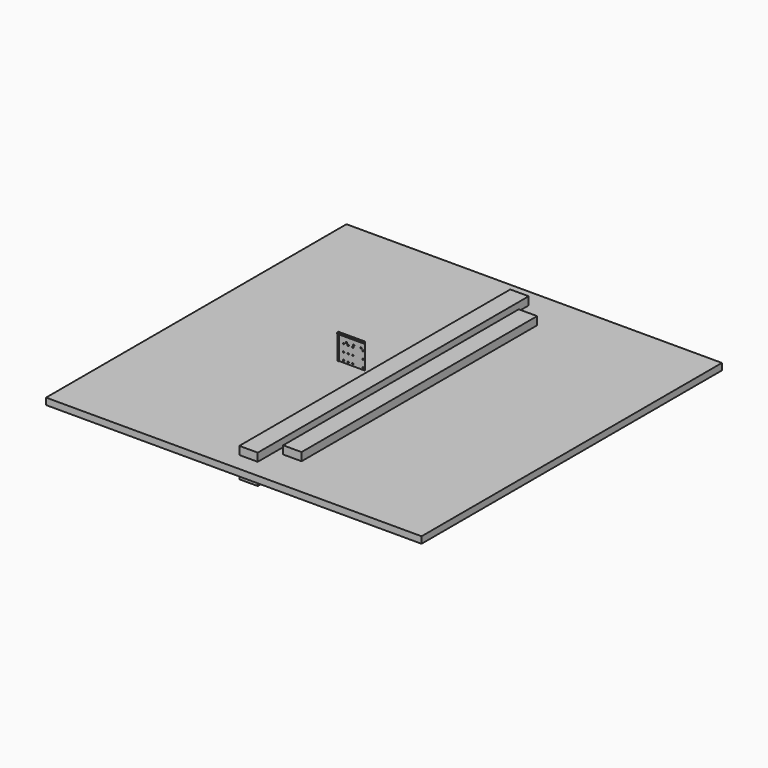
from build123d import *

# Parameters (mm, degrees)
F0_W     = 50
F0_H     = 80
F1_DEPTH = 460
F2_DEPTH = 400
F3_R     = 1.85
F3_W     = 2.75
F3_H     = 65.8975437433
F3_W_2   = 20.0489750504
F3_H_2   = 2.75
F4_DEPTH = 1.5
F5_DEPTH = 5
F6_DEPTH = 3.5
F7_W     = 1020
F7_H     = 1020
F8_DEPTH = 18


with BuildPart() as f1:
    # F0 (on Front) → F1 (new body, symmetric)
    with BuildSketch(Plane.XZ):
        Rectangle(F0_W, F0_H)
    extrude(amount=F1_DEPTH, both=True)


with BuildPart() as f2:
    # F0 (on Front) → F2 (new body, symmetric)
    with BuildSketch(Plane.XZ):
        with Locations((71.0044652224, 0)):
            Rectangle(F0_W, F0_H)
    extrude(amount=F2_DEPTH, both=True)


with BuildPart() as f4:
    # F3 (on Front) → F4 (new body)
    with BuildSketch(Plane.XZ):
        Polygon((-121.2795429826, 25.1443590969), (-71.0295429826, 25.1443590969), (-71.0295429826, 90.7919028401), (-71.0295429826, 91.0419028401), (-121.2795429826, 91.0419028401), align=None)
        with Locations((-108.5295429826, 30.7919028401)):
            Circle(F3_R, mode=Mode.SUBTRACT)
        with Locations((-96.0295429826, 30.7919028401)):
            Circle(F3_R, mode=Mode.SUBTRACT)
        with Locations((-108.5295429826, 50.7919028401)):
            Circle(F3_R, mode=Mode.SUBTRACT)
        with Locations((-96.0295429826, 50.7919028401)):
            Circle(F3_R, mode=Mode.SUBTRACT)
        with Locations((-83.5295429826, 30.7919028401)):
            Circle(F3_R, mode=Mode.SUBTRACT)
        with Locations((-83.5295429826, 50.7919028401)):
            Circle(F3_R, mode=Mode.SUBTRACT)
        with Locations((-108.5295429826, 70.7919028401)):
            Circle(F3_R, mode=Mode.SUBTRACT)
        with Locations((-101.0295429826, 75.7919028401)):
            Circle(F3_R, mode=Mode.SUBTRACT)
        with Locations((-96.0295429826, 70.7919028401)):
            Circle(F3_R, mode=Mode.SUBTRACT)
        with Locations((-83.5295429826, 70.7919028401)):
            Circle(F3_R, mode=Mode.SUBTRACT)
        with Locations((-81.0295429826, 75.7919028401)):
            Circle(F3_R, mode=Mode.SUBTRACT)
        Polygon((-71.0295429826, 90.7919028401), (-71.0295429826, 25.1443590969), (-50.9805679321, 25.1443590969), (-50.9805679321, 91.0419028401), (-71.0295429826, 91.0419028401), align=None)
        with Locations((-56.0295429826, 30.3744599223)):
            Circle(F3_R, mode=Mode.SUBTRACT)
        with Locations((-56.0295429826, 50.7919028401)):
            Circle(F3_R, mode=Mode.SUBTRACT)
        with Locations((-61.0295429826, 75.7919028401)):
            Circle(F3_R, mode=Mode.SUBTRACT)
        with Locations((-56.0295429826, 70.7919028401)):
            Circle(F3_R, mode=Mode.SUBTRACT)
        with Locations((-122.6545429826, 58.0931309685)):
            Rectangle(F3_W, F3_H)
        Polygon((-121.2795429826, 91.0419028401), (-71.0295429826, 91.0419028401), (-71.0295429826, 93.7919028401), (-124.0295429826, 93.7919028401), (-124.0295429826, 91.0419028401), align=None)
        with Locations((-61.0050554574, 92.4169028401)):
            Rectangle(F3_W_2, F3_H_2)
    extrude(amount=F4_DEPTH)

    # F3 (on Front) → F5 (join)
    with BuildSketch(Plane.XZ):
        Polygon((-121.2795429826, 91.0419028401), (-71.0295429826, 91.0419028401), (-71.0295429826, 93.7919028401), (-124.0295429826, 93.7919028401), (-124.0295429826, 91.0419028401), align=None)
        with Locations((-61.0050554574, 92.4169028401)):
            Rectangle(F3_W_2, F3_H_2)
    extrude(amount=F5_DEPTH)

    # F3 (on Front) → F6 (join)
    with BuildSketch(Plane.XZ):
        with Locations((-122.6545429826, 58.0931309685)):
            Rectangle(F3_W, F3_H)
    extrude(amount=F6_DEPTH)


with BuildPart() as f8:
    # F7 (on Top) → F8 (new body)
    with BuildSketch(Plane.XY):
        Rectangle(F7_W, F7_H)
    extrude(amount=F8_DEPTH)


solid = Compound([f1.part, f2.part, f4.part, f8.part])
